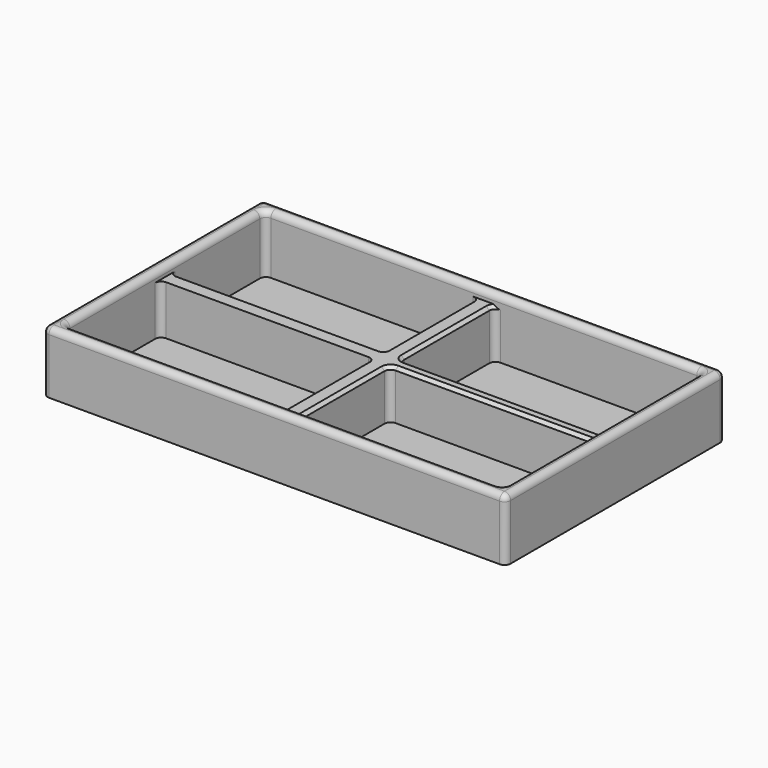
from build123d import *

# Parameters (mm, degrees)
F0_W         = 150
F0_H         = 88.883145673
F1_DEPTH     = 20
F2_W         = 142
F2_H         = 80.883145673
F3_DEPTH     = 19
F5_DEPTH     = 16
F6_R         = 1.99999
F7_T1_DEPTH  = 63.6293265809
F7_T3_DEPTH  = 34.4415928365
F7_T5_DEPTH  = 34.4415928365
F7_T8_ANGLE  = 90
F7_T10_ANGLE = 90
F7_T14_ANGLE = 163.703254406
F7_T19_ANGLE = 163.703254406
F7_T24_ANGLE = 163.703254406
F7_T29_ANGLE = 163.703254406


# Not quite as in the source:
# - a fillet or chamfer that OpenCascade refuses, or shapes differently, is made with other operations: its cross-section is extruded or revolved along the edge and cut away or added
# - a fillet or chamfer is up to 0.001 mm smaller than in the source, because OpenCascade refuses the exact size
# - a feature names something its author has since deleted; it is built from what else it names


with BuildPart() as f1:
    # F0 (on Top) → F1 (new body)
    with BuildSketch(Plane.XY):
        Rectangle(F0_W, F0_H)
    extrude(amount=F1_DEPTH)

    # F2 (on face) → F3 (cut)
    with BuildSketch(Plane.XY.offset(20)):
        Rectangle(F2_W, F2_H)
    extrude(amount=-F3_DEPTH, mode=Mode.SUBTRACT)

    # F4 (on face) → F5 (join)
    with BuildSketch(Plane.XY.offset(1)):
        Polygon((3.3706934191, -2), (71, -2), (71, 2), (3.3706934191, 2), (3.3706934191, 40.4415728365), (-1.4311365085, 40.4415728365), (-1.4311365085, 2), (-71, 2), (-71, -2), (-1.4311365085, -2), (-1.4311365085, -40.4415728365), (3.3706934191, -40.4415728365), align=None)
    extrude(amount=F5_DEPTH)

    # F6 (radius 2 in the source; OpenCascade refuses exactly that, so slightly less here)
    f6_edges = [f1.edges().sort_by_distance(p)[0] for p in [
        (-75, 0, 20),
        (0, 44.441573, 20),
        (0, -44.441573, 20),
        (75, 0, 20),
        (-75, -44.441573, 10),
        (-75, 44.441573, 10),
        (75, -44.441573, 10),
        (75, 44.441573, 10),
        (0, 44.441573, 0),
        (-71, -40.441573, 10.5),
        (-71, 40.441573, 10.5),
        (71, -40.441573, 10.5),
        (71, 40.441573, 10.5),
        (71, 2, 9),
        (71, -2, 9),
        (71, 0, 20),
        (0, 40.441573, 20),
        (0, -40.441573, 20),
        (-71, 0, 20),
        (-1.431137, 2, 9),
        (3.370693, 2, 9),
        (-1.431137, -2, 9),
        (-1.431137, 40.441573, 9),
        (3.370693, 40.441573, 9),
        (-71, -2, 9),
        (-71, 2, 9),
        (3.370693, -40.441573, 9),
        (-1.431137, -40.441573, 9),
        (3.370693, -2, 9),
    ]]
    fillet(f6_edges, radius=F6_R)

    # F7: chamfer of 1 on 6 edges, made by hand

    # F7_s2 → F7_t1 (cut)
    with BuildSketch(Plane.YZ.offset(5.3706834191)):
        Polygon((1, 17), (2, 16), (2, 17), align=None)
        Polygon((-1, 17), (-2, 16), (-2, 17), align=None)
    extrude(amount=F7_T1_DEPTH, mode=Mode.SUBTRACT)

    # F7_s4 → F7_t3 (cut)
    with BuildSketch(Plane.XZ.offset(3.99999)):
        Polygon((2.3706934191, 17), (3.3706934191, 16), (3.3706934191, 17), align=None)
    extrude(amount=F7_T3_DEPTH, mode=Mode.SUBTRACT)

    # F7_s6 → F7_t5 (cut)
    with BuildSketch(Plane.XZ.offset(-38.4415828365)):
        Polygon((2.3706934191, 17), (3.3706934191, 16), (3.3706934191, 17), align=None)
    extrude(amount=F7_T5_DEPTH, mode=Mode.SUBTRACT)

    # F7_s7 → F7_t8 (revolve, cut)
    with BuildSketch(Plane.XZ.offset(3.99999)):
        Polygon((2.3706934191, 17), (3.3706934191, 16), (3.3706934191, 17), align=None)
    revolve(axis=Axis((5.3706834191, -3.99999, 17), (0, 0, -1)), revolution_arc=F7_T8_ANGLE, mode=Mode.SUBTRACT)

    # F7_s9 → F7_t10 (revolve, cut)
    with BuildSketch(Plane.YZ.offset(5.3706834191)):
        Polygon((1, 17), (2, 16), (2, 17), align=None)
    revolve(axis=Axis((5.3706834191, 3.99999, 17), (0, 0, -1)), revolution_arc=F7_T10_ANGLE, mode=Mode.SUBTRACT)


with BuildPart() as f7_tool12:
    # F7_s13 → F7_t14 (revolve)
    with BuildSketch(Plane(origin=(-9.930856522, 33.9680428578, 0), x_dir=(0, 0, 1), z_dir=(0.2806121914, -0.9598212323, 0))):
        Polygon((17, -18.9420627796), (16, -17.9420627796), (17, -17.9420627796), align=None)
    revolve(axis=Axis((5.3706834191, 38.4415828365, 17), (0, 0, 1)), revolution_arc=F7_T14_ANGLE)

    split(bisect_by=Plane.XZ.offset(-40.4415728365), keep=Keep.TOP)


with BuildPart() as f1_1:
    add(f1.part)

    # F7_t11: cut F7_tool12
    add(f7_tool12.part, mode=Mode.SUBTRACT)


with BuildPart() as f7_tool17:
    # F7_s18 → F7_t19 (revolve)
    with BuildSketch(Plane(origin=(-9.930856522, -33.9680428578, 0), x_dir=(0, 0, 1), z_dir=(0.2806121914, 0.9598212323, 0))):
        Polygon((17, 18.9420627796), (16, 17.9420627796), (17, 17.9420627796), align=None)
    revolve(axis=Axis((5.3706834191, -38.4415828365, 17), (0, 0, -1)), revolution_arc=F7_T19_ANGLE)

    split(bisect_by=Plane.XZ.offset(40.4415728365), keep=Keep.BOTTOM)


with BuildPart() as f1_2:
    add(f1_1.part)

    # F7_t16: cut F7_tool17
    add(f7_tool17.part, mode=Mode.SUBTRACT)


with BuildPart() as f7_tool22:
    # F7_s23 → F7_t24 (revolve)
    with BuildSketch(Plane(origin=(62.4893808118, 18.2693208905, 0), x_dir=(0, 0, 1), z_dir=(-0.9598212323, -0.2806121914, 0))):
        Polygon((17, -26.201509346), (16, -25.201509346), (17, -25.201509346), align=None)
    revolve(axis=Axis((69.00001, -3.99999, 17), (0, 0, 1)), revolution_arc=F7_T24_ANGLE)

    split(bisect_by=Plane.YZ.offset(71), keep=Keep.BOTTOM)


with BuildPart() as f1_3:
    add(f1_2.part)

    # F7_t21: cut F7_tool22
    add(f7_tool22.part, mode=Mode.SUBTRACT)


with BuildPart() as f7_tool27:
    # F7_s28 → F7_t29 (revolve)
    with BuildSketch(Plane(origin=(62.4893808118, -18.2693208905, 0), x_dir=(0, 0, 1), z_dir=(-0.9598212323, 0.2806121914, 0))):
        Polygon((16, 25.201509346), (17, 26.201509346), (17, 25.201509346), align=None)
    revolve(axis=Axis((69.00001, 3.99999, 17), (0, 0, -1)), revolution_arc=F7_T29_ANGLE)

    split(bisect_by=Plane.YZ.offset(71), keep=Keep.BOTTOM)


with BuildPart() as f1_4:
    add(f1_3.part)

    # F7_t26: cut F7_tool27
    add(f7_tool27.part, mode=Mode.SUBTRACT)


solid = f1_4.part
